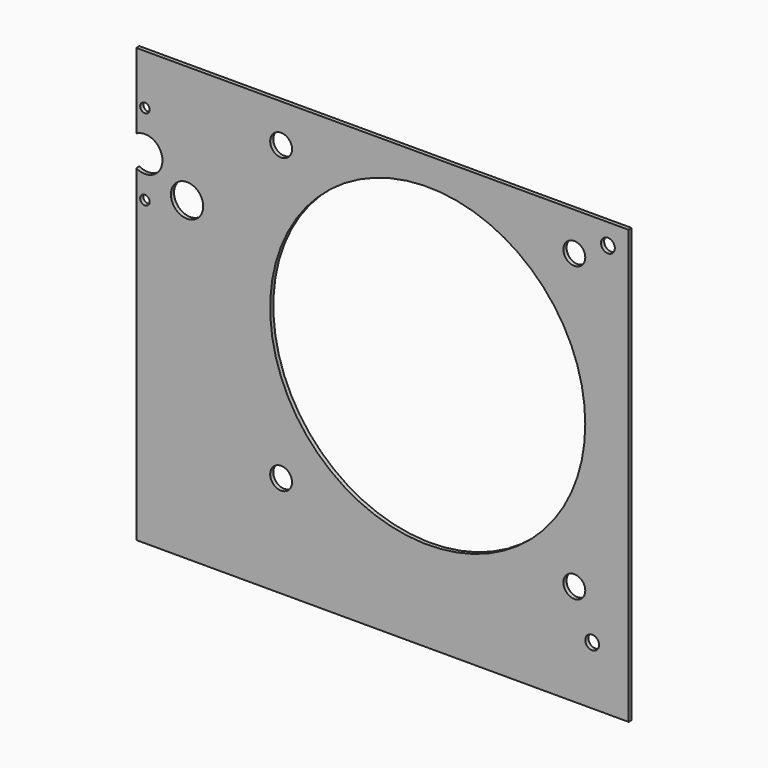
from build123d import *

# Parameters (mm, degrees)
F0_R     = 2.778
F0_R_2   = 1.75
F0_R_3   = 1.2
F0_R_4   = 4.1
F0_R_5   = 40
F1_DEPTH = 1


# Not quite as in the source:
# - a feature names something its author has since deleted; it is built from what else it names


with BuildPart() as f1:
    # F0 (on Front) → F1 (new body)
    with BuildSketch(Plane.XZ):
        with BuildLine():
            Line((-62.5, 28.1318609125), (-62.5, -55))
            Line((-62.5, -55), (62.5, -55))
            Line((62.5, -55), (62.5, 55))
            Line((62.5, 55), (-62.5, 55))
            Line((-62.5, 55), (-62.5, 35.8681390875))
            ThreePointArc((-62.5, 35.8681390875), (-58.0625349165, 35.8465893984), (-55.85, 32))
            ThreePointArc((-55.85, 32), (-58.0625349165, 28.1534106016), (-62.5, 28.1318609125))
        make_face()
        with Locations((-25.722, -29.222)):
            Circle(F0_R, mode=Mode.SUBTRACT)
        with Locations((53.25, -40.25)):
            Circle(F0_R_2, mode=Mode.SUBTRACT)
        with Locations((48.722, -29.222)):
            Circle(F0_R, mode=Mode.SUBTRACT)
        with Locations((-60.3, 21.7)):
            Circle(F0_R_3, mode=Mode.SUBTRACT)
        with Locations((-49.6, 25.1)):
            Circle(F0_R_4, mode=Mode.SUBTRACT)
        with Locations((-60.3, 42.3)):
            Circle(F0_R_3, mode=Mode.SUBTRACT)
        with Locations((-25.722, 45.222)):
            Circle(F0_R, mode=Mode.SUBTRACT)
        with Locations((11.5, 8)):
            Circle(F0_R_5, mode=Mode.SUBTRACT)
        with Locations((48.722, 45.222)):
            Circle(F0_R, mode=Mode.SUBTRACT)
        with Locations((57.25, 49.75)):
            Circle(F0_R_2, mode=Mode.SUBTRACT)
    extrude(amount=F1_DEPTH)


solid = f1.part
